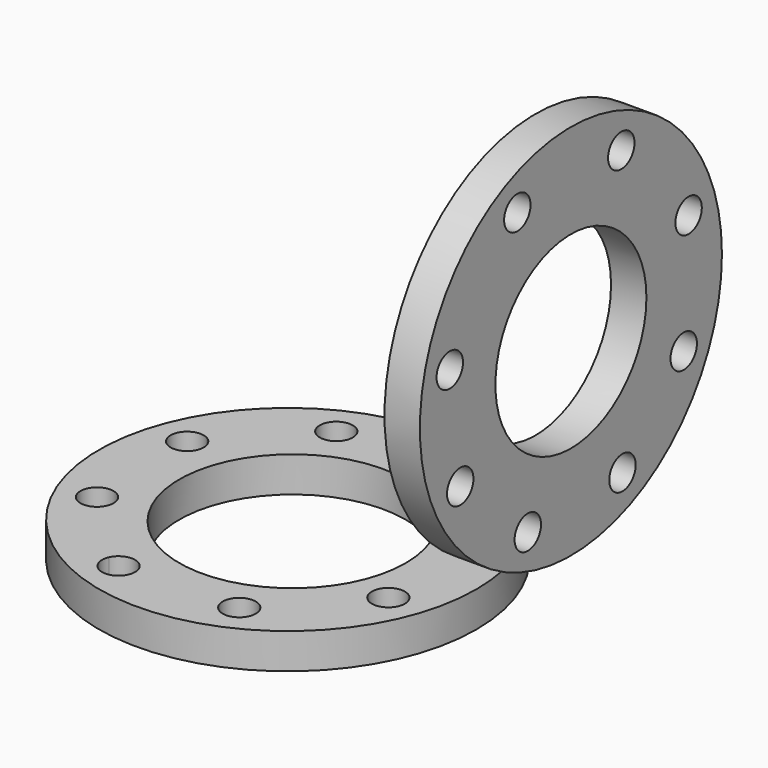
from build123d import *

# Parameters (mm, degrees)
F0_R     = 127
F0_R_2   = 76.2
F1_DEPTH = 23.8125
F4_R     = 127
F4_R_2   = 11.1125
F4_R_3   = 63.5
F5_DEPTH = 23.8125


# Not quite as in the source:
# - the program builds the solid bodies; features that only make, move or delete a surface that nothing else refers to are left out


with BuildPart() as f1:
    # F0 (on Top) → F1 (new body)
    with BuildSketch(Plane.XY):
        Circle(F0_R)
        with BuildLine():
            ThreePointArc((101.9958548396, 34.7946514115), (106.4448025713, 17.6495395986), (107.942049028, 0))
            ThreePointArc((107.942049028, 0), (106.9823052387, -14.1489647287), (104.120656465, -28.03871913))
            ThreePointArc((104.120656465, -28.03871913), (106.9261709336, -31.8112513898), (107.920677619, -36.4062342556))
            ThreePointArc((107.920677619, -36.4062342556), (104.5734800406, -44.3553055569), (96.548306946, -47.5156952454))
            ThreePointArc((96.548306946, -47.5156952454), (78.4010780991, -72.9221605187), (53.5731929065, -91.8532595192))
            ThreePointArc((53.5731929065, -91.8532595192), (53.7604643817, -93.0183920588), (53.8231237491, -94.1968139884))
            ThreePointArc((53.8231237491, -94.1968139884), (45.9011634738, -104.8414423292), (33.4302126102, -100.3092296601))
            ThreePointArc((33.4302126102, -100.3092296601), (3.751342164, -104.7733707892), (-25.9754714164, -100.6405193108))
            ThreePointArc((-25.9754714164, -100.6405193108), (-40.6110553172, -107.0944371963), (-46.5346943911, -92.2363124052))
            ThreePointArc((-46.5346943911, -92.2363124052), (-70.0459417897, -74.9510413572), (-87.8779817622, -51.8517405051))
            ThreePointArc((-87.8779817622, -51.8517405051), (-104.373234586, -47.1747160498), (-96.6430601698, -31.8707189585))
            ThreePointArc((-96.6430601698, -31.8707189585), (-101.5542755055, -3.3533286372), (-98.4775871181, 25.4198459422))
            ThreePointArc((-98.4775871181, 25.4198459422), (-107.24989988, 40.2086140993), (-91.0220503046, 45.893509257))
            ThreePointArc((-91.0220503046, 45.893509257), (-74.7387890105, 70.0605525565), (-52.4291016529, 88.8080438613))
            ThreePointArc((-52.4291016529, 88.8080438613), (-47.5764375285, 104.187385169), (-32.4760746868, 98.5259780812))
            ThreePointArc((-32.4760746868, 98.5259780812), (-3.176203782, 104.5828081894), (26.6409177774, 102.1115963588))
            ThreePointArc((26.6409177774, 102.1115963588), (39.1421597741, 107.5786171554), (47.5187342556, 96.808177619))
            ThreePointArc((47.5187342556, 96.808177619), (47.4814140774, 95.8982061001), (47.3697042146, 94.994346671))
            ThreePointArc((47.3697042146, 94.994346671), (73.3279865341, 77.8154449532), (93.0935679461, 53.7682231459))
            ThreePointArc((93.0935679461, 53.7682231459), (101.6542879107, 50.9491757425), (105.3093139884, 42.7106237491))
            ThreePointArc((105.3093139884, 42.7106237491), (104.4475334195, 38.4198886844), (101.9958548396, 34.7946514115))
        make_face(mode=Mode.SUBTRACT)
        with BuildLine():
            ThreePointArc((104.120656465, -28.03871913), (106.9823052387, -14.1489647287), (107.942049028, 0))
            ThreePointArc((107.942049028, 0), (106.4448025713, 17.6495395986), (101.9958548396, 34.7946514115))
            ThreePointArc((101.9958548396, 34.7946514115), (84.1366190041, 37.9904401586), (93.0935679461, 53.7682231459))
            ThreePointArc((93.0935679461, 53.7682231459), (73.3279865341, 77.8154449532), (47.3697042146, 94.994346671))
            ThreePointArc((47.3697042146, 94.994346671), (32.7975359141, 86.2979467686), (26.6409177774, 102.1115963588))
            ThreePointArc((26.6409177774, 102.1115963588), (-3.176203782, 104.5828081894), (-32.4760746868, 98.5259780812))
            ThreePointArc((-32.4760746868, 98.5259780812), (-31.8198229818, 96.4054594778), (-31.5981237491, 94.1968139884))
            ThreePointArc((-31.5981237491, 94.1968139884), (-39.9275435721, 83.4384627681), (-52.4291016529, 88.8080438613))
            ThreePointArc((-52.4291016529, 88.8080438613), (-74.7387890105, 70.0605525565), (-91.0220503046, 45.893509257))
            ThreePointArc((-91.0220503046, 45.893509257), (-87.1183376815, 41.8463315189), (-85.695677619, 36.4062342556))
            ThreePointArc((-85.695677619, 36.4062342556), (-89.5646859475, 27.9789283603), (-98.4775871181, 25.4198459422))
            ThreePointArc((-98.4775871181, 25.4198459422), (-101.5542755055, -3.3533286372), (-96.6430601698, -31.8707189585))
            ThreePointArc((-96.6430601698, -31.8707189585), (-87.2576589404, -34.031004894), (-83.0843139884, -42.7106237491))
            ThreePointArc((-83.0843139884, -42.7106237491), (-84.3554299555, -47.8715167502), (-87.8779817622, -51.8517405051))
            ThreePointArc((-87.8779817622, -51.8517405051), (-70.0459417897, -74.9510413572), (-46.5346943911, -92.2363124052))
            ThreePointArc((-46.5346943911, -92.2363124052), (-34.067950377, -85.9444726915), (-25.2937342556, -96.808177619))
            ThreePointArc((-25.2937342556, -96.808177619), (-25.4654959739, -98.7544309683), (-25.9754714164, -100.6405193108))
            ThreePointArc((-25.9754714164, -100.6405193108), (3.751342164, -104.7733707892), (33.4302126102, -100.3092296601))
            ThreePointArc((33.4302126102, -100.3092296601), (38.4092677124, -83.9505467415), (53.5731929065, -91.8532595192))
            ThreePointArc((53.5731929065, -91.8532595192), (78.4010780991, -72.9221605187), (96.548306946, -47.5156952454))
            ThreePointArc((96.548306946, -47.5156952454), (86.45091108, -32.3794879152), (104.120656465, -28.03871913))
        make_face()
        with Locations((3.167049028, 0)):
            Circle(F0_R_2, mode=Mode.SUBTRACT)
    extrude(amount=F1_DEPTH)


with BuildPart() as f5:
    # F4 (on offset) → F5 (new body)
    with BuildSketch(Plane.YZ.offset(190.5)):
        with Locations((0, 191.315561533)):
            Circle(F4_R)
        with Locations((-36.2507900525, 93.011539003)):
            Circle(F4_R_2, mode=Mode.SUBTRACT)
        with Locations((-93.0804328953, 143.21323688)):
            Circle(F4_R_2, mode=Mode.SUBTRACT)
        with Locations((43.3518492061, 95.9299347572)):
            Circle(F4_R_2, mode=Mode.SUBTRACT)
        with Locations((94.8888080869, 146.8868014237)):
            Circle(F4_R_2, mode=Mode.SUBTRACT)
        with Locations((-101.882713284, 215.7637385384)):
            Circle(F4_R_2, mode=Mode.SUBTRACT)
        with Locations((-45.0610448925, 285.9057452636)):
            Circle(F4_R_2, mode=Mode.SUBTRACT)
        with Locations((0, 191.315561533)):
            Circle(F4_R_3, mode=Mode.SUBTRACT)
        with Locations((98.9754160548, 225.6909545021)):
            Circle(F4_R_2, mode=Mode.SUBTRACT)
        with Locations((42.3611944988, 287.1452533077)):
            Circle(F4_R_2, mode=Mode.SUBTRACT)
    extrude(amount=-F5_DEPTH)


solid = Compound([f1.part, f5.part])
